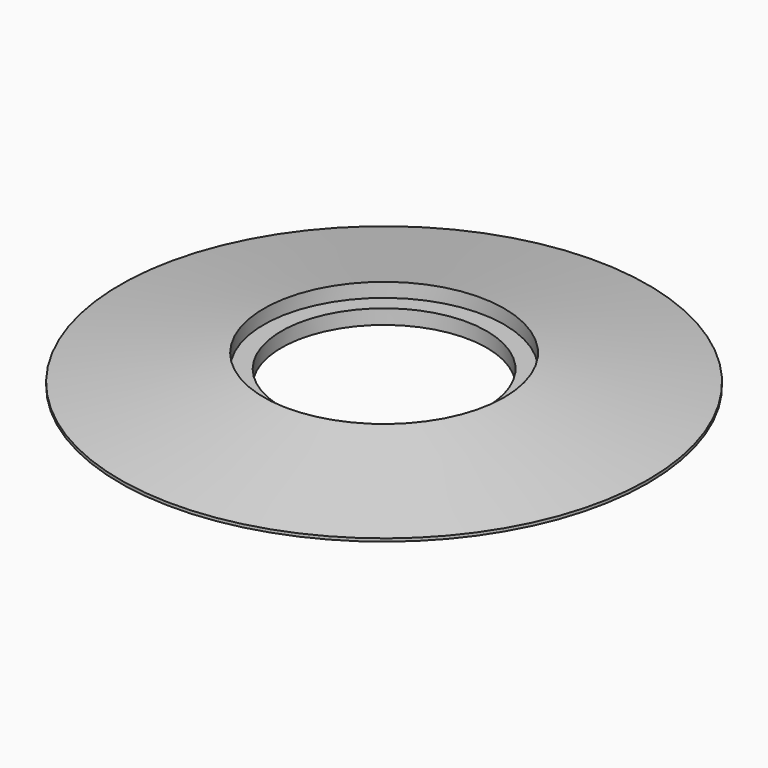
from build123d import *

# Parameters (mm, degrees)
F0_R     = 45
F0_R_2   = 20.5
F1_DEPTH = 5
F0_R_3   = 17.5
F2_DEPTH = 2.5


# Not quite as in the source:
# - a fillet or chamfer that OpenCascade refuses, or shapes differently, is made with other operations: its cross-section is extruded or revolved along the edge and cut away or added


with BuildPart() as f1:
    # F0 (on Top) → F1 (new body)
    with BuildSketch(Plane.XY):
        Circle(F0_R)
        Circle(F0_R_2, mode=Mode.SUBTRACT)
    extrude(amount=F1_DEPTH)

    # F0 (on Top) → F2 (join)
    with BuildSketch(Plane.XY):
        Circle(F0_R_2)
        Circle(F0_R_3, mode=Mode.SUBTRACT)
    extrude(amount=F2_DEPTH)

    # F3: chamfer of 25 x 4.5 on 1 edges, made by hand

    # F3_s1 → F3_t2 (revolve, cut)
    with BuildSketch(Plane.XZ):
        Polygon((45, 0.5), (20, 5), (45, 5), align=None)
    revolve(axis=Axis((0, 0, 5), (0, 0, 1)), mode=Mode.SUBTRACT)


solid = f1.part
